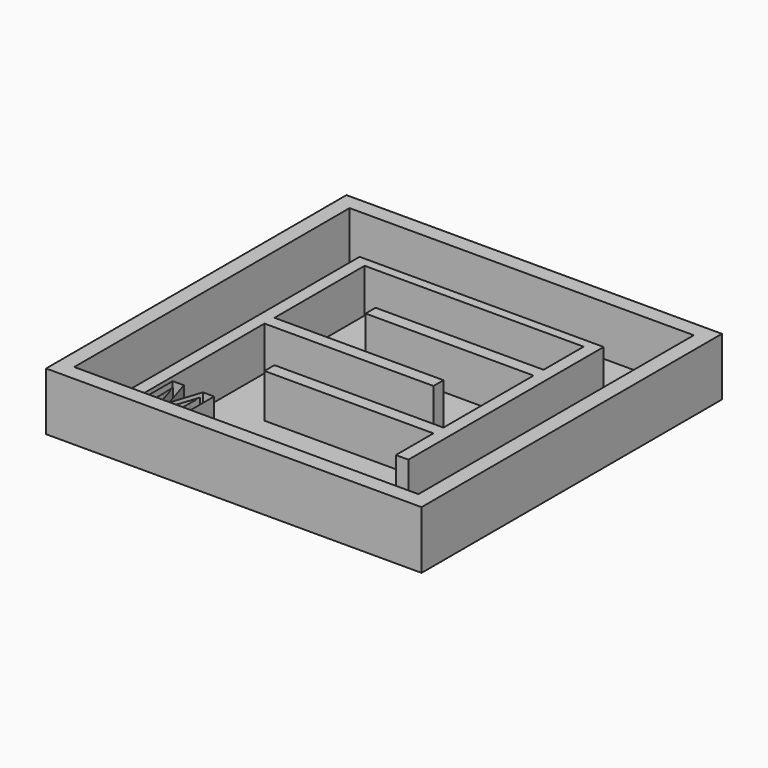
from build123d import *

# Parameters (mm, degrees)
F0_W         = 38.1
F0_H         = 38.1
F1_DEPTH     = 0.79375
F2_W         = 38.1
F2_H         = 38.1
F2_W_2       = 34.925
F2_H_2       = 34.925
F3_DEPTH     = 5.08
F4_R         = 1.27
F5_DEPTH     = 0.396875
F4_W         = 17.0465118896
F4_H         = 1.27
F4_W_2       = 17.145
F6_DEPTH     = 4.445
F7_TEXT_SIZE = 5.51008812
F8_DEPTH     = 4.445


# Not quite as in the source:
# - Text() gives the source's letters only with a copy of the font that has no kerning and outlines rounded to 1/6400 em; it was checked with that copy


with BuildPart() as f1:
    # F0 (on Top) → F1 (new body)
    with BuildSketch(Plane.XY):
        with Locations((4.5851375908, -2.053696575)):
            Rectangle(F0_W, F0_H)
    extrude(amount=F1_DEPTH)

    # F2 (on face) → F3 (join)
    with BuildSketch(Plane.XY.offset(0.79375)):
        with Locations((4.5851375908, -2.053696575)):
            Rectangle(F2_W, F2_H)
        with Locations((4.5851375908, -2.053696575)):
            Rectangle(F2_W_2, F2_H_2, mode=Mode.SUBTRACT)
    extrude(amount=F3_DEPTH)

    # F4 (on face) → F5 (cut)
    with BuildSketch(Plane.XY.offset(0.79375)):
        with Locations((-10.3373624092, -16.6561957449)):
            Circle(F4_R)
        with Locations((13.2783399895, 6.836303425)):
            Circle(F4_R)
    extrude(amount=-F5_DEPTH, mode=Mode.SUBTRACT)

    # F4 (on face) → F6 (join)
    with BuildSketch(Plane.XY.offset(0.79375)):
        Polygon((-7.7973624092, 10.328803425), (-7.7973624092, -19.516196575), (-6.5273624092, -19.516196575), (-6.5273624092, -3.323696575), (-6.5273624092, -2.053696575), (-6.5273624092, 9.376303425), (15.6976375908, 9.376303425), (15.6976375908, 9.058803425), (15.6976375908, 4.296303425), (15.6976375908, 3.026303425), (15.6976375908, -8.403696575), (15.6976375908, -9.673696575), (15.6976375908, -14.436196575), (16.9676375908, -14.436196575), (16.9676375908, 9.376303425), (16.9676375908, 10.328803425), (-6.5273624092, 10.328803425), align=None)
        with Locations((7.174381646, 3.661303425)):
            Rectangle(F4_W, F4_H)
        with Locations((2.0451375908, -2.688696575)):
            Rectangle(F4_W_2, F4_H)
        with Locations((7.1251375908, -9.038696575)):
            Rectangle(F4_W_2, F4_H)
    extrude(amount=F6_DEPTH)

    # F7 (on face) → F8 (join)
    with BuildSketch(Plane.XY.offset(0.79375)):
        with Locations((-6.5273624092, -19.516196575)):
            Text('M', F7_TEXT_SIZE, font='Open Sans', font_style=FontStyle.BOLD, text_align=(TextAlign.LEFT, TextAlign.BOTTOM))
    extrude(amount=F8_DEPTH)


solid = f1.part
